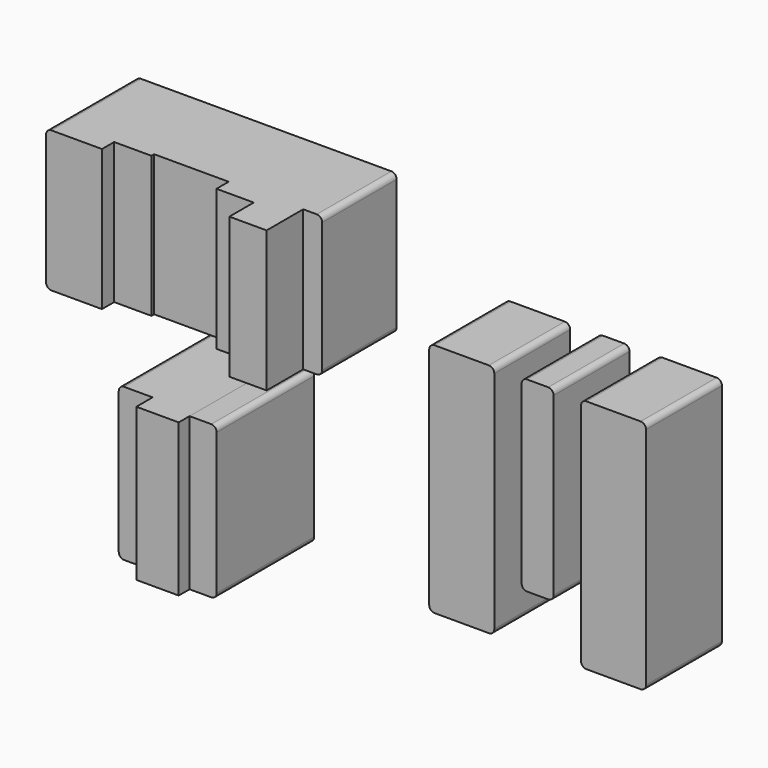
from build123d import *

# Parameters (mm, degrees)
F0_W      = 60.96
F0_H      = 220.98
F1_DEPTH  = 88.9
F0_W_2    = 29.972
F0_H_2    = 175.006
F2_R      = 5.08
F2_2_R    = 5.08
F2_3_R    = 5.08
F3_R      = 5.08
F0_W_3    = 52.3875
F0_H_3    = 132.08
F4_DEPTH  = 104.775
F0_W_4    = 34.925
F5_DEPTH  = 90.5002
F0_W_5    = 69.85
F6_DEPTH  = 87.3252
F7_DEPTH  = 101.6
F8_DEPTH  = 130.175
F0_W_6    = 17.78
F9_DEPTH  = 87.3252
F0_W_7    = 31.75
F0_H_4    = 142.875
F10_DEPTH = 107.95
F0_W_8    = 39.6875
F11_DEPTH = 127
F0_W_9    = 25.4
F12_DEPTH = 114.3
F13_R     = 5.08
F13_2_R   = 5.08
F13_3_R   = 5.08


with BuildPart() as f1:
    # F0 (on Front) → F1 (new body)
    with BuildSketch(Plane.XZ):
        with Locations((453.0725, -245.11)):
            Rectangle(F0_W, F0_H)
    extrude(amount=F1_DEPTH)

    # F2
    f2_edges = [f1.edges().sort_by_distance(p)[0] for p in [
        (483.5525, -44.45, -134.62),
        (422.5925, -44.45, -134.62),
        (422.5925, -44.45, -355.6),
        (483.5525, -44.45, -355.6),
    ]]
    fillet(f2_edges, radius=F2_R)


with BuildPart() as f1b:
    # F0 (on Front) → F1, piece 2 (new body)
    with BuildSketch(Plane.XZ):
        with Locations((595.3125, -245.11)):
            Rectangle(F0_W, F0_H)
    extrude(amount=F1_DEPTH)

    # F2#2
    f2_2_edges = [f1b.edges().sort_by_distance(p)[0] for p in [
        (625.7925, -44.45, -134.62),
        (564.8325, -44.45, -134.62),
        (564.8325, -44.45, -355.6),
        (625.7925, -44.45, -355.6),
    ]]
    fillet(f2_2_edges, radius=F2_2_R)


with BuildPart() as f1c:
    # F0 (on Front) → F1, piece 3 (new body)
    with BuildSketch(Plane.XZ):
        with Locations((524.1925, -222.123)):
            Rectangle(F0_W_2, F0_H_2)
    extrude(amount=F1_DEPTH)

    # F2#3
    f2_3_edges = [f1c.edges().sort_by_distance(p)[0] for p in [
        (539.1785, -44.45, -134.62),
        (509.2065, -44.45, -309.626),
        (539.1785, -44.45, -309.626),
    ]]
    fillet(f2_3_edges, radius=F2_3_R)

    # F3
    f3_edges = [f1c.edges().sort_by_distance(p)[0] for p in [
        (509.2065, -44.45, -134.62),
    ]]
    fillet(f3_edges, radius=F3_R)


with BuildPart() as f4:
    # F0 (on Front) → F4 (new body)
    with BuildSketch(Plane.XZ):
        with Locations((102.39375, -129.54)):
            Rectangle(F0_W_3, F0_H_3)
    extrude(amount=F4_DEPTH)

    # F0 (on Front) → F5 (join)
    with BuildSketch(Plane.XZ):
        with Locations((146.05, -129.54)):
            Rectangle(F0_W_4, F0_H_3)
    extrude(amount=F5_DEPTH)

    # F0 (on Front) → F6 (join)
    with BuildSketch(Plane.XZ):
        with Locations((198.4375, -129.54)):
            Rectangle(F0_W_5, F0_H_3)
    extrude(amount=F6_DEPTH)

    # F0 (on Front) → F7 (join)
    with BuildSketch(Plane.XZ):
        with Locations((250.825, -129.54)):
            Rectangle(F0_W_4, F0_H_3)
    extrude(amount=F7_DEPTH)

    # F0 (on Front) → F8 (join)
    with BuildSketch(Plane.XZ):
        with Locations((285.75, -129.54)):
            Rectangle(F0_W_4, F0_H_3)
    extrude(amount=F8_DEPTH)

    # F0 (on Front) → F9 (join)
    with BuildSketch(Plane.XZ):
        with Locations((312.1025, -129.54)):
            Rectangle(F0_W_6, F0_H_3)
    extrude(amount=F9_DEPTH)

    # F13
    f13_edges = [f4.edges().sort_by_distance(p)[0] for p in [
        (320.9925, -43.6626, -63.5),
        (76.2, -52.3875, -63.5),
        (320.9925, -43.6626, -195.58),
        (76.2, -52.3875, -195.58),
    ]]
    fillet(f13_edges, radius=F13_R)


with BuildPart() as f10:
    # F0 (on Front) → F10 (new body)
    with BuildSketch(Plane.XZ):
        with Locations((162.7124, -322.2625)):
            Rectangle(F0_W_7, F0_H_4)
    extrude(amount=F10_DEPTH)

    # F0 (on Front) → F11 (join)
    with BuildSketch(Plane.XZ):
        with Locations((198.43115, -322.2625)):
            Rectangle(F0_W_8, F0_H_4)
    extrude(amount=F11_DEPTH)

    # F13#2
    f13_2_edges = [f10.edges().sort_by_distance(p)[0] for p in [
        (146.8374, -53.975, -250.825),
        (146.8374, -53.975, -393.7),
    ]]
    fillet(f13_2_edges, radius=F13_2_R)


with BuildPart() as f12:
    # F0 (on Front) → F12 (new body)
    with BuildSketch(Plane.XZ):
        with Locations((230.9749, -322.2625)):
            Rectangle(F0_W_9, F0_H_4)
    extrude(amount=F12_DEPTH)

    # F13#3
    f13_3_edges = [f12.edges().sort_by_distance(p)[0] for p in [
        (243.6749, -57.15, -250.825),
        (243.6749, -57.15, -393.7),
    ]]
    fillet(f13_3_edges, radius=F13_3_R)


solid = Compound([f1.part, f1b.part, f1c.part, f4.part, f10.part, f12.part])
